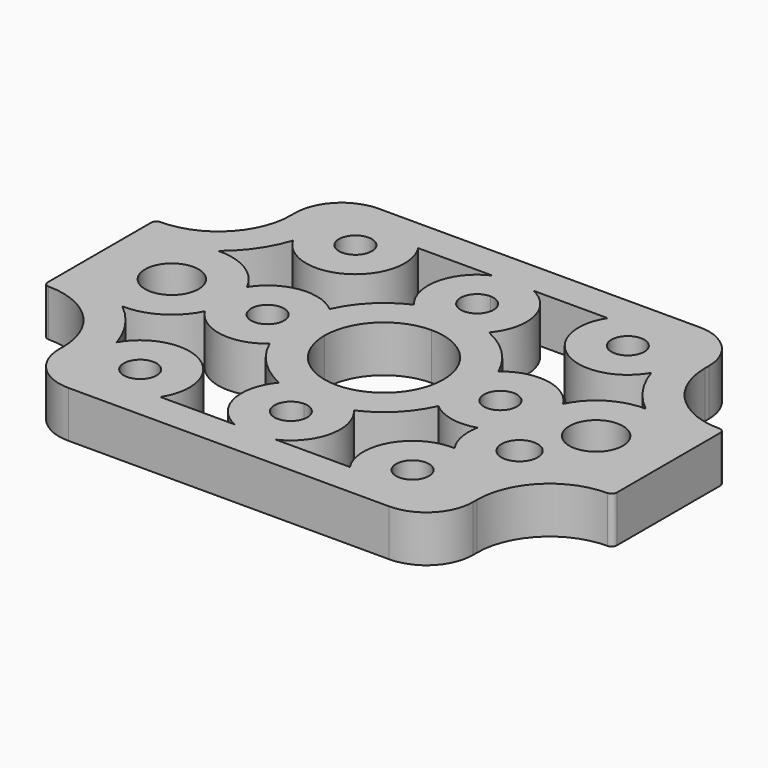
from build123d import *

# Parameters (mm, degrees)
F0_R     = 3.175
F0_R_2   = 3.5
F1_DEPTH = 9


# Not quite as in the source:
# - ends of sketch curves that miss each other by under 0.0002 mm in the source are joined


with BuildPart() as f1:
    # F0 (on Top) → F1 (new body)
    with BuildSketch(Plane.XY):
        with BuildLine():
            Line((0, 25.675), (0, 37.5))
            Line((0, 37.5), (-31, 37.5))
            ThreePointArc((-31, 37.5), (-37.3639610307, 34.8639610307), (-40, 28.5))
            Line((-40, 28.5), (-40, 27.5))
            ThreePointArc((-40, 27.5), (-44.1005050634, 17.6005050634), (-54, 13.5))
            ThreePointArc((-54, 13.5), (-54.7071067812, 13.2071067812), (-55, 12.5))
            Line((-55, 12.5), (-55, 0))
            Line((-55, 0), (-46.175, 0))
            ThreePointArc((-46.175, 0), (-41, 5.175), (-35.825, 0))
            Line((-35.825, 0), (-25.675, 0))
            ThreePointArc((-25.675, 0), (-22.5, 3.175), (-19.325, 0))
            Line((-19.325, 0), (-11.5, 0))
            ThreePointArc((-11.5, 0), (-8.1317279836, 8.1317279836), (0, 11.5))
            Line((0, 11.5), (0, 19.325))
            ThreePointArc((0, 19.325), (-3.175, 22.5), (0, 25.675))
        make_face()
        with BuildLine():
            ThreePointArc((-30.5652871781, 5.0672249135), (-34.9739264655, 9.9119341078), (-41.3041070016, 11.5960130619))
            ThreePointArc((-41.3041070016, 11.5960130619), (-37.2403076286, 15.9572441931), (-34.6146149846, 21.3089299951))
            ThreePointArc((-34.6146149846, 21.3089299951), (-21.4024086548, 17.845567287), (-18.3122078194, 31.1500001161))
            Line((-18.3122078194, 31.1500001161), (-3.987873, 31.15))
            ThreePointArc((-3.987873, 31.15), (-9.3036595822, 24.5414561908), (-7.2431808946, 16.31437509))
            ThreePointArc((-7.2431808946, 16.31437509), (-12.6218560442, 12.6218560442), (-16.3143749324, 7.24318097))
            ThreePointArc((-16.3143749324, 7.24318097), (-23.9376990029, 9.4158720561), (-30.5652871781, 5.0672249135))
        make_face(mode=Mode.SUBTRACT)
        with Locations((-26.324893, 26)):
            Circle(F0_R, mode=Mode.SUBTRACT)
        with BuildLine():
            ThreePointArc((0, -11.5), (-8.1317279836, -8.1317279836), (-11.5, 0))
            Line((-11.5, 0), (-19.325, 0))
            ThreePointArc((-19.325, 0), (-22.5, -3.175), (-25.675, 0))
            Line((-25.675, 0), (-35.825, 0))
            ThreePointArc((-35.825, 0), (-41, -5.175), (-46.175, 0))
            Line((-46.175, 0), (-55, 0))
            Line((-55, 0), (-55, -12.5))
            ThreePointArc((-55, -12.5), (-54.7071067812, -13.2071067812), (-54, -13.5))
            ThreePointArc((-54, -13.5), (-44.1005050634, -17.6005050634), (-40, -27.5))
            Line((-40, -27.5), (-40, -28.5))
            ThreePointArc((-40, -28.5), (-37.3639610307, -34.8639610307), (-31, -37.5))
            Line((-31, -37.5), (0, -37.5))
            Line((0, -37.5), (0, -25.675))
            ThreePointArc((0, -25.675), (-3.175, -22.5), (0, -19.325))
            Line((0, -19.325), (0, -11.5))
        make_face()
        with Locations((-26.324893, -26)):
            Circle(F0_R, mode=Mode.SUBTRACT)
        with BuildLine():
            ThreePointArc((-34.6146149846, -21.3089299951), (-37.2403076286, -15.9572441931), (-41.304107024, -11.59601303))
            ThreePointArc((-41.304107024, -11.59601303), (-34.9739264655, -9.9119341078), (-30.5652871781, -5.0672249135))
            ThreePointArc((-30.5652871781, -5.0672249135), (-23.9376990029, -9.4158720561), (-16.31437509, -7.2431808946))
            ThreePointArc((-16.31437509, -7.2431808946), (-12.6218560442, -12.6218560442), (-7.24318097, -16.3143749324))
            ThreePointArc((-7.24318097, -16.3143749324), (-9.3036595822, -24.5414561908), (-3.9878728667, -31.1499997109))
            Line((-3.9878728667, -31.1499997109), (-18.312208, -31.15))
            ThreePointArc((-18.312208, -31.15), (-21.4024086548, -17.845567287), (-34.6146149846, -21.3089299951))
        make_face(mode=Mode.SUBTRACT)
        with BuildLine():
            Line((19.325, 0), (11.5, 0))
            ThreePointArc((11.5, 0), (8.1317279836, -8.1317279836), (0, -11.5))
            Line((0, -11.5), (0, -19.325))
            ThreePointArc((0, -19.325), (2.2450640303, -20.2549359697), (3.175, -22.5))
            ThreePointArc((3.175, -22.5), (2.2450640303, -24.7450640303), (0, -25.675))
            Line((0, -25.675), (0, -37.5))
            Line((0, -37.5), (31, -37.5))
            ThreePointArc((31, -37.5), (37.3639610307, -34.8639610307), (40, -28.5))
            Line((40, -28.5), (40, -27.5))
            ThreePointArc((40, -27.5), (44.1005050634, -17.6005050634), (54, -13.5))
            ThreePointArc((54, -13.5), (54.7071067812, -13.2071067812), (55, -12.5))
            Line((55, -12.5), (55, 0))
            Line((55, 0), (46.175, 0))
            ThreePointArc((46.175, 0), (41, -5.175), (35.825, 0))
            Line((35.825, 0), (25.675, 0))
            ThreePointArc((25.675, 0), (22.5, -3.175), (19.325, 0))
        make_face()
        with Locations((26.324893, -26)):
            Circle(F0_R, mode=Mode.SUBTRACT)
        with BuildLine():
            ThreePointArc((7.24318097, -16.3143749324), (12.6218560442, -12.6218560442), (16.3143749324, -7.24318097))
            ThreePointArc((16.3143749324, -7.24318097), (20.5869660419, -9.3309123924), (25.3363869117, -9.0928837168))
            ThreePointArc((25.3363869117, -9.0928837168), (25.3425465049, -12.93806398), (26.8204236463, -16.4878985664))
            ThreePointArc((26.8204236463, -16.4878985664), (18.0864944073, -21.2193710008), (18.3122078194, -31.1500001161))
            Line((18.3122078194, -31.1500001161), (3.987872, -31.15))
            ThreePointArc((3.987872, -31.15), (9.3036594849, -24.5414566343), (7.24318097, -16.3143749324))
        make_face(mode=Mode.SUBTRACT)
        with Locations((35, -11)):
            Circle(F0_R_2, mode=Mode.SUBTRACT)
        with BuildLine():
            Line((31, 37.5), (0, 37.5))
            Line((0, 37.5), (0, 25.675))
            ThreePointArc((0, 25.675), (2.2450640303, 24.7450640303), (3.175, 22.5))
            ThreePointArc((3.175, 22.5), (2.2450640303, 20.2549359697), (0, 19.325))
            Line((0, 19.325), (0, 11.5))
            ThreePointArc((0, 11.5), (8.1317279836, 8.1317279836), (11.5, 0))
            Line((11.5, 0), (19.325, 0))
            ThreePointArc((19.325, 0), (22.5, 3.175), (25.675, 0))
            Line((25.675, 0), (35.825, 0))
            ThreePointArc((35.825, 0), (41, 5.175), (46.175, 0))
            Line((46.175, 0), (55, 0))
            Line((55, 0), (55, 12.5))
            ThreePointArc((55, 12.5), (54.7071067812, 13.2071067812), (54, 13.5))
            ThreePointArc((54, 13.5), (44.1005050634, 17.6005050634), (40, 27.5))
            Line((40, 27.5), (40, 28.5))
            ThreePointArc((40, 28.5), (37.3639610307, 34.8639610307), (31, 37.5))
        make_face()
        with BuildLine():
            ThreePointArc((30.5652870625, 5.0672250393), (23.9376990029, 9.4158720561), (16.31437509, 7.2431808946))
            ThreePointArc((16.31437509, 7.2431808946), (12.6218560442, 12.6218560442), (7.24318097, 16.3143749324))
            ThreePointArc((7.24318097, 16.3143749324), (9.3036594849, 24.5414566343), (3.987872042, 31.1500000911))
            Line((3.987872042, 31.1500000911), (18.312208, 31.15))
            ThreePointArc((18.312208, 31.15), (21.4024086548, 17.845567287), (34.6146148363, 21.3089300926))
            ThreePointArc((34.6146148363, 21.3089300926), (37.2403076286, 15.9572441931), (41.304107024, 11.59601303))
            ThreePointArc((41.304107024, 11.59601303), (34.9739264655, 9.9119341078), (30.5652870625, 5.0672250393))
        make_face(mode=Mode.SUBTRACT)
        with Locations((26.324893, 26)):
            Circle(F0_R, mode=Mode.SUBTRACT)
    extrude(amount=F1_DEPTH)


solid = f1.part
